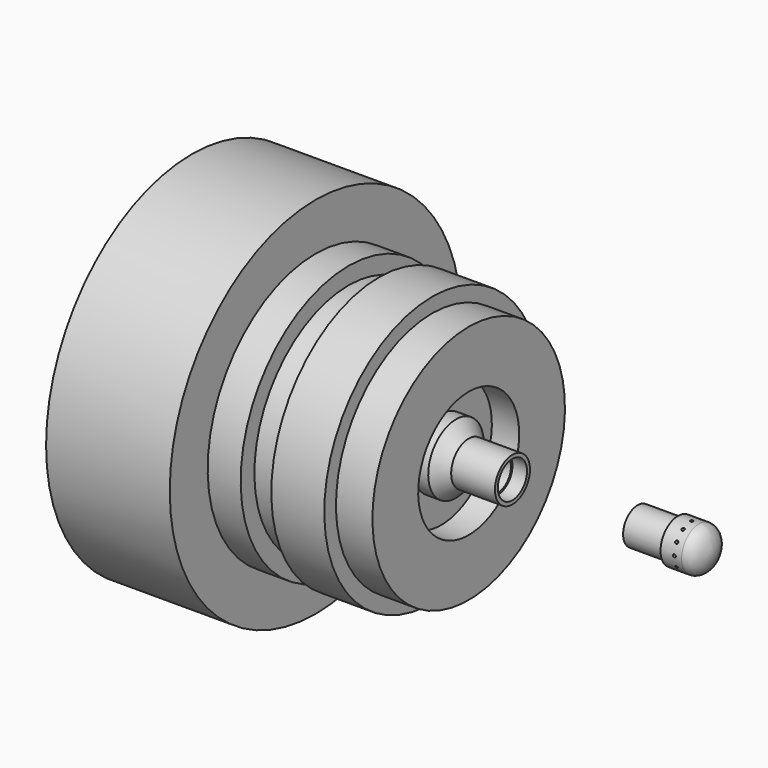
from build123d import *

# Parameters (mm, degrees)
F2_R            = 0.2
F3_DEPTH        = 25
F3_COPIES_COUNT = 12


# Not quite as in the source:
# - a pattern or mirror of a feature is missing from the dataset's text; its kind, count and spacing are read off the source's solid


with BuildPart() as f1:
    # F0 (on Front) → F1 (revolve)
    with BuildSketch(Plane.XZ):
        with BuildLine():
            Line((9.0803319924, 2.5), (3.5476123448, 2.5))
            Line((3.5476123448, 2.5), (3.5476123448, 1.5))
            Line((3.5476123448, 1.5), (12.0749778994, 1.5))
            Line((12.0749778994, 1.5), (12.9762688279, 0))
            Line((12.9762688279, 0), (13.9762688279, 0))
            add(Edge.make_bspline(
                [(13.9762688279, 0), (13.9762688279, 3), (11.9762688279, 3)],
                knots=[4.7123889804, 4.7123889804, 4.7123889804, 6.2831853072, 6.2831853072, 6.2831853072], degree=2, weights=[1, 0.7071067812, 1]))
            Line((11.9762688279, 3), (9.0803319924, 3))
            Line((9.0803319924, 3), (9.0803319924, 2.5))
        make_face()
    revolve(axis=Axis((10.6589230162, 0, 0), (1, 0, 0)))

    # F2 (on Front) → F3 (cut)
    with BuildSketch(Plane.XZ):
        with Locations((10.9762688279, 0)):
            Circle(F2_R)
    f3 = extrude(amount=F3_DEPTH, mode=Mode.SUBTRACT)

    # F3_copies: F3 ×12 about axis
    f3_copies_axis = Axis((0, 0, 0), (1, 0, 0))
    for i in range(1, F3_COPIES_COUNT):
        add(f3.rotate(f3_copies_axis, i * 360 / F3_COPIES_COUNT), mode=Mode.SUBTRACT)


with BuildPart() as f5:
    # F4 (on Front) → F5 (revolve)
    with BuildSketch(Plane.XZ):
        Polygon((-15.6235943586, 2.5), (-13.6235943586, 2.5), (-13.6235943586, 3), (-19.6235943586, 3), (-21.3735943586, 4.75), (-23.3735943586, 4.75), (-23.3735943586, 8.656449616), (-19.6235943586, 8.656449616), (-19.6235943586, 16.5), (-24.6235943586, 16.5), (-24.6235943586, 18.5), (-31.8873989864, 18.5), (-31.8873989864, 16.15), (-36.0873989864, 16.15), (-36.0873989864, 18.5), (-40.6128289125, 18.5), (-40.6128289125, 25), (-57.5714183428, 25), (-57.5714183428, 0), (-29.3572743084, 0), (-29.3572743084, 2.25), (-15.6235943586, 2.25), align=None)
    revolve(axis=Axis((-42.681645602, 0, 0), (-1, 0, 0)))


solid = Compound([f1.part, f5.part])
